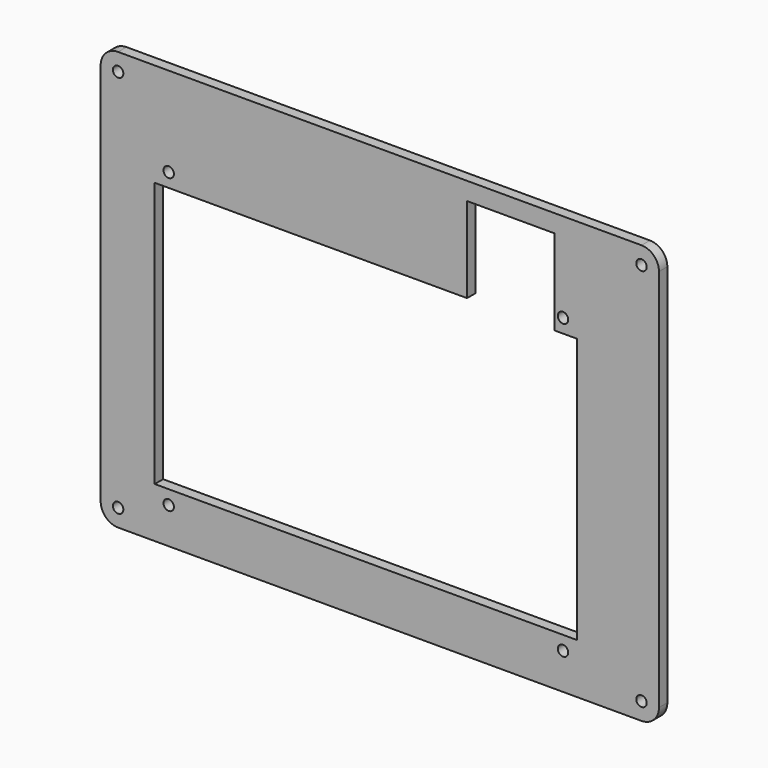
from build123d import *

# Parameters (mm, degrees)
F1_DEPTH = 3
F2_R     = 1.5
F3_DEPTH = 25
F4_R     = 1.5
F5_DEPTH = 25
F6_W     = 121
F6_H     = 76
F6_R     = 1.5
F7_DEPTH = 3
F8_W     = 25
F8_H     = 24.5
F9_DEPTH = 3


# Not quite as in the source:
# - a feature names something its author has since deleted; it is built from what else it names


with BuildPart() as f1:
    # F0 (on Front) → F1 (new body)
    with BuildSketch(Plane.XZ):
        with BuildLine():
            Line((-75, -60), (75, -60))
            ThreePointArc((75, -60), (78.5355339059, -58.5355339059), (80, -55))
            Line((80, -55), (80, 55))
            ThreePointArc((80, 55), (78.5355339059, 58.5355339059), (75, 60))
            Line((75, 60), (-75, 60))
            ThreePointArc((-75, 60), (-78.5355339059, 58.5355339059), (-80, 55))
            Line((-80, 55), (-80, -55))
            ThreePointArc((-80, -55), (-78.5355339059, -58.5355339059), (-75, -60))
        make_face()
    extrude(amount=F1_DEPTH)

    # F2 (on Front) → F3 (cut)
    with BuildSketch(Plane.XZ):
        with Locations((-75, 55)):
            Circle(F2_R)
        with Locations((75, 55)):
            Circle(F2_R)
        with Locations((75, -55)):
            Circle(F2_R)
        with Locations((-75, -55)):
            Circle(F2_R)
    extrude(amount=F3_DEPTH, mode=Mode.SUBTRACT)

    # F4 (on Front) → F5 (cut)
    with BuildSketch(Plane.XZ):
        with Locations((52.5, 34.4)):
            Circle(F4_R)
    extrude(amount=F5_DEPTH, mode=Mode.SUBTRACT)

    # F6 (on face) → F7 (cut)
    with BuildSketch(Plane.XZ.offset(3)):
        with Locations((-4, -7.6)):
            Rectangle(F6_W, F6_H)
        with Locations((52.5, 34.4)):
            Circle(F6_R)
        with Locations((-60.5, 34.4)):
            Circle(F6_R)
        with Locations((-60.5, -49.6)):
            Circle(F6_R)
        with Locations((52.5, -49.6)):
            Circle(F6_R)
    extrude(amount=-F7_DEPTH, mode=Mode.SUBTRACT)

    # F8 (on face) → F9 (cut)
    with BuildSketch(Plane.XZ.offset(3)):
        with Locations((37.5, 42.65)):
            Rectangle(F8_W, F8_H)
    extrude(amount=-F9_DEPTH, mode=Mode.SUBTRACT)


solid = f1.part
